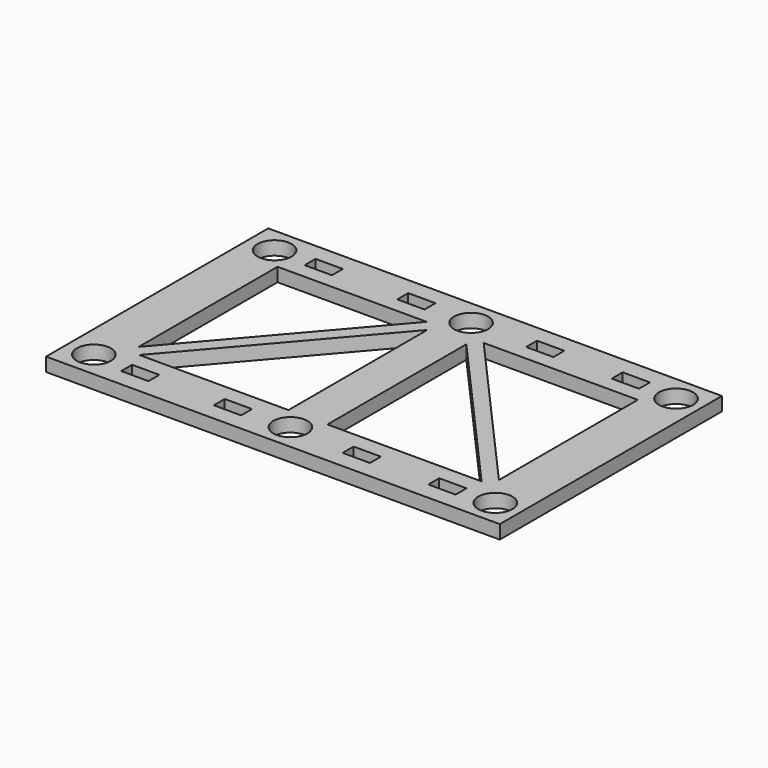
from build123d import *

# Parameters (mm, degrees)
F0_W     = 66.5
F0_H     = 40.7
F0_R     = 2.5
F0_W_2   = 4
F0_H_2   = 2
F0_W_3   = 23.1688134372
F0_H_3   = 26.9576453138
F0_W_4   = 23.9260006735
F1_DEPTH = 2
F0_H_4   = 1.6511697322
F0_H_5   = 1.6511703735
F2_E4_W  = 35.5458655395
F2_E4_H  = 2
F3_DEPTH = 1
F4_E5_W  = 36.0439752121
F4_E5_H  = 2
F5_DEPTH = 1


with BuildPart() as f1:
    # F0 (on Top) → F1 (new body)
    with BuildSketch(Plane.XY):
        with Locations((-26.3848016039, -10.9677366539)):
            Rectangle(F0_W, F0_H)
        with Locations((-55.6704513729, -27.5134705007)):
            Circle(F0_R, mode=Mode.SUBTRACT)
        with Locations((-48.6798131391, -27.7539507372)):
            Rectangle(F0_W_2, F0_H_2, mode=Mode.SUBTRACT)
        with Locations((-35.1007831245, -27.7539507372)):
            Rectangle(F0_W_2, F0_H_2, mode=Mode.SUBTRACT)
        with Locations((-26.8697291613, -27.5134705007)):
            Circle(F0_R, mode=Mode.SUBTRACT)
        with Locations((-16.2120581007, -27.7539507372)):
            Rectangle(F0_W_2, F0_H_2, mode=Mode.SUBTRACT)
        with Locations((-3.6603234261, -27.7539507372)):
            Rectangle(F0_W_2, F0_H_2, mode=Mode.SUBTRACT)
        with Locations((3.1705482397, -27.5134705007)):
            Circle(F0_R, mode=Mode.SUBTRACT)
        with Locations((-55.6704513729, 5.5923270993)):
            Circle(F0_R, mode=Mode.SUBTRACT)
        with Locations((-48.6798131391, 5.8541836441)):
            Rectangle(F0_W_2, F0_H_2, mode=Mode.SUBTRACT)
        with Locations((-41.2725005299, -10.8643159037)):
            Rectangle(F0_W_3, F0_H_3, mode=Mode.SUBTRACT)
        with Locations((-35.1007831245, 5.8541836441)):
            Rectangle(F0_W_2, F0_H_2, mode=Mode.SUBTRACT)
        with Locations((-26.8697291613, 5.5923270993)):
            Circle(F0_R, mode=Mode.SUBTRACT)
        with Locations((-12.0121349685, -10.8643159037)):
            Rectangle(F0_W_4, F0_H_3, mode=Mode.SUBTRACT)
        with Locations((-16.2120581007, 5.8541836441)):
            Rectangle(F0_W_2, F0_H_2, mode=Mode.SUBTRACT)
        with Locations((-3.6603234261, 5.8541836441)):
            Rectangle(F0_W_2, F0_H_2, mode=Mode.SUBTRACT)
        with Locations((3.1705482397, 5.5923270993)):
            Circle(F0_R, mode=Mode.SUBTRACT)
    extrude(amount=F1_DEPTH)

    # F2_E4 (on explicit) → F3 (join, symmetric)
    with BuildSketch(Plane(origin=(-52.8569072485, -24.3431385607, 0), x_dir=(0.6518005142, 0.7583904599, 0), z_dir=(0.7583904599, -0.6518005142, 0))):
        with Locations((17.7729327698, 1)):
            Rectangle(F2_E4_W, F2_E4_H)
    extrude(amount=F3_DEPTH, both=True)

    # F4_E5 (on explicit) → F5 (join, symmetric)
    with BuildSketch(Plane(origin=(-23.9751353052, 2.6145067532, 0), x_dir=(0.6638002754, -0.7479098838, 0), z_dir=(-0.7479098838, -0.6638002754, 0))):
        with Locations((18.0219876061, 1)):
            Rectangle(F4_E5_W, F4_E5_H)
    extrude(amount=F5_DEPTH, both=True)


with BuildPart() as f1b:
    # F0 (on Top) → F1, piece 2 (new body)
    with BuildSketch(Plane.XY):
        with Locations((-3.6603234261, 39.867881812)):
            Rectangle(F0_W_2, F0_H_4)
    extrude(amount=F1_DEPTH)


with BuildPart() as f1c:
    # F0 (on Top) → F1, piece 3 (new body)
    with BuildSketch(Plane.XY):
        with Locations((-3.6603234261, -61.797210648)):
            Rectangle(F0_W_2, F0_H_5)
    extrude(amount=F1_DEPTH)


solid = f1.part
